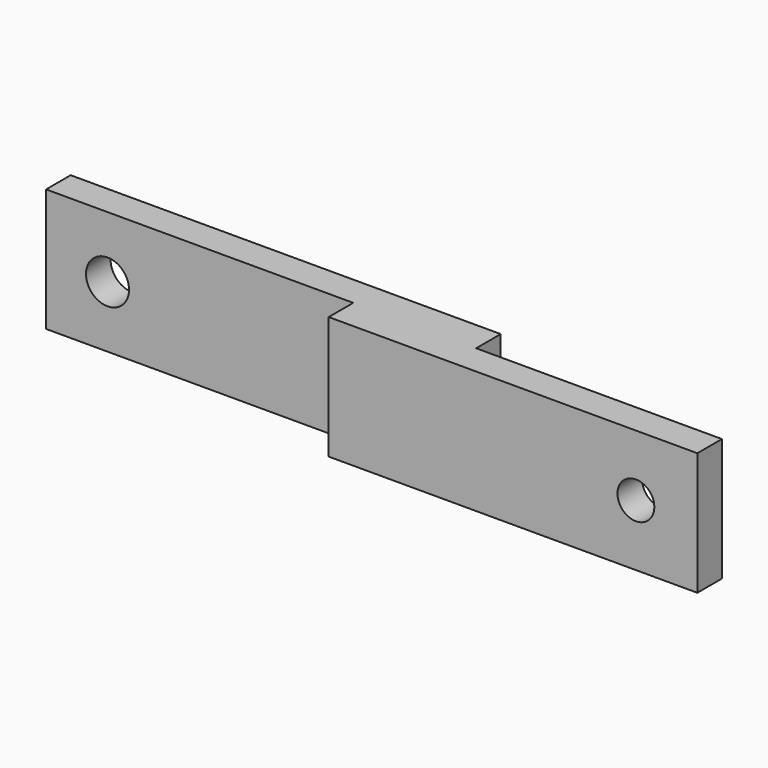
from build123d import *

# Parameters (mm, degrees)
F0_W     = 10
F0_H     = 40
F1_DEPTH = 140
F2_R     = 7
F3_DEPTH = 10.001
F4_W     = 80
F4_H     = 40
F4_R     = 6
F4_W_2   = 40
F5_DEPTH = 10
F7_DEPTH = 10


# Not quite as in the source:
# - a feature names something its author has since deleted; it is built from what else it names


with BuildPart() as f1:
    # F0 (on Right) → F1 (new body)
    with BuildSketch(Plane.YZ):
        Rectangle(F0_W, F0_H)
    extrude(amount=-F1_DEPTH)

    # F2 (on face) → F3 (cut, through all)
    with BuildSketch(Plane.XZ.offset(5)):
        with Locations((-120, 0)):
            Circle(F2_R)
    extrude(amount=-F3_DEPTH, mode=Mode.SUBTRACT)

    # F4 (on face) → F5 (join)
    with BuildSketch(Plane.XZ.offset(5)):
        with Locations((40, 0)):
            Rectangle(F4_W, F4_H)
        with Locations((60, 0)):
            Circle(F4_R, mode=Mode.SUBTRACT)
        with Locations((-20, 0)):
            Rectangle(F4_W_2, F4_H)
    extrude(amount=F5_DEPTH)

    # F6 (on face) → F7 (cut, through all)
    with BuildSketch(Plane(origin=(0, 5, 0), x_dir=(-1, 0, 0), z_dir=(0, 1, 0))):
        Polygon((15, -20), (0, -5), (0, -20), align=None)
    extrude(amount=-F7_DEPTH, mode=Mode.SUBTRACT)


solid = f1.part
